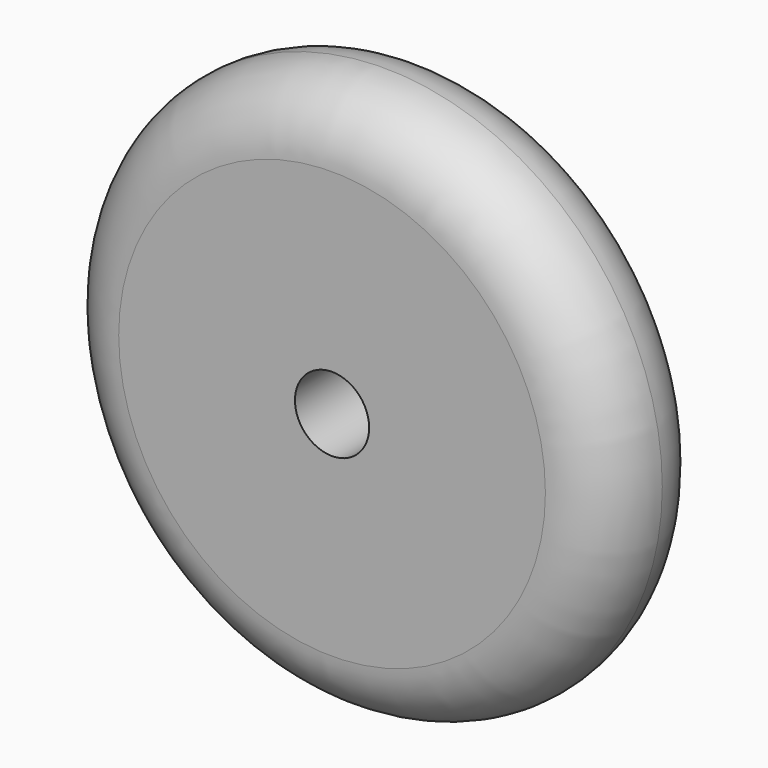
from build123d import *

# Parameters (mm, degrees)
F0_R     = 30
F1_DEPTH = 14
F2_R     = 6.99999
F4_D     = 8
F4_DEPTH = 100
F4_TIP   = 2.4034424761


# Not quite as in the source:
# - a fillet or chamfer is up to 0.001 mm smaller than in the source, because OpenCascade refuses the exact size


with BuildPart() as f1:
    # F0 (on Front) → F1 (new body)
    with BuildSketch(Plane.XZ):
        Circle(F0_R)
    extrude(amount=F1_DEPTH)

    # F2 (radius 7 in the source; OpenCascade refuses exactly that, so slightly less here)
    f2_edges = [f1.edges().sort_by_distance(p)[0] for p in [
        (-30, -14, 0),
        (-30, 0, 0),
    ]]
    fillet(f2_edges, radius=F2_R)

    # F4
    with Locations(Plane(origin=(0, 0, 0), x_dir=(-1, 0, 0), z_dir=(0, 1, 0))):
        with Locations((0, 0)):
            Hole(F4_D / 2, depth=F4_DEPTH)
            with Locations((0, 0, -(F4_DEPTH + F4_TIP / 2))):  # 118° drill point
                Cone(0, F4_D / 2, F4_TIP, mode=Mode.SUBTRACT)


solid = f1.part
